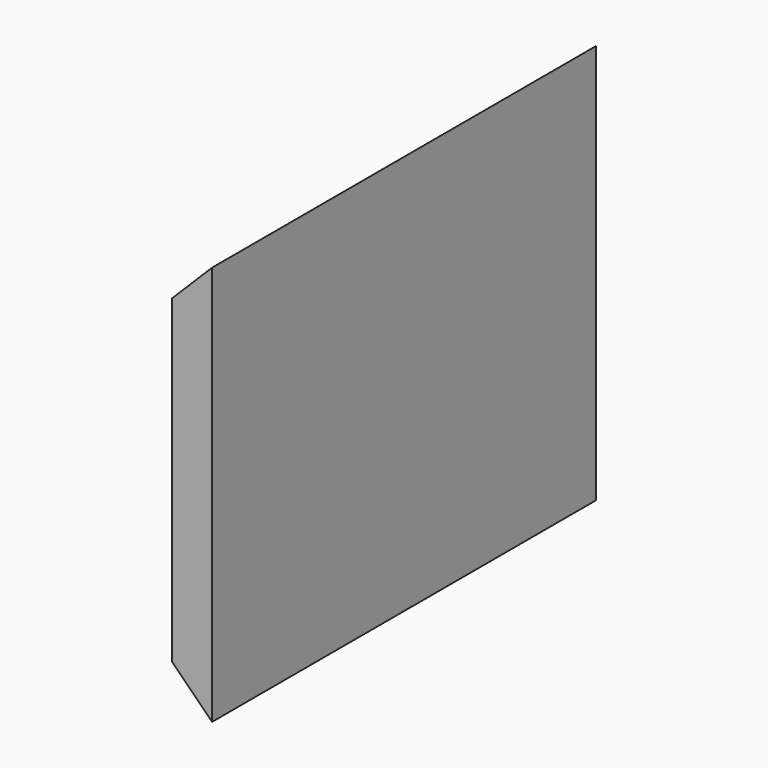
from build123d import *

# Parameters (mm, degrees)
F0_W     = 25
F0_H     = 250
F1_DEPTH = 300
F2_SIZE  = 24.99999
F3_SIZE  = 24.99999


# Not quite as in the source:
# - a fillet or chamfer is up to 0.001 mm smaller than in the source, because OpenCascade refuses the exact size


with BuildPart() as f1:
    # F0 (on Front) → F1 (new body)
    with BuildSketch(Plane.XZ):
        with Locations((12.5, 125)):
            Rectangle(F0_W, F0_H)
    extrude(amount=F1_DEPTH)

    # F2 (size 25 in the source; OpenCascade refuses exactly that, so slightly less here)
    f2_edges = [f1.edges().sort_by_distance(p)[0] for p in [
        (0, -150, 250),
    ]]
    chamfer(f2_edges, length=F2_SIZE)

    # F3 (size 25 in the source; OpenCascade refuses exactly that, so slightly less here)
    f3_edges = [f1.edges().sort_by_distance(p)[0] for p in [
        (0, -150, 0),
    ]]
    chamfer(f3_edges, length=F3_SIZE)


solid = f1.part
